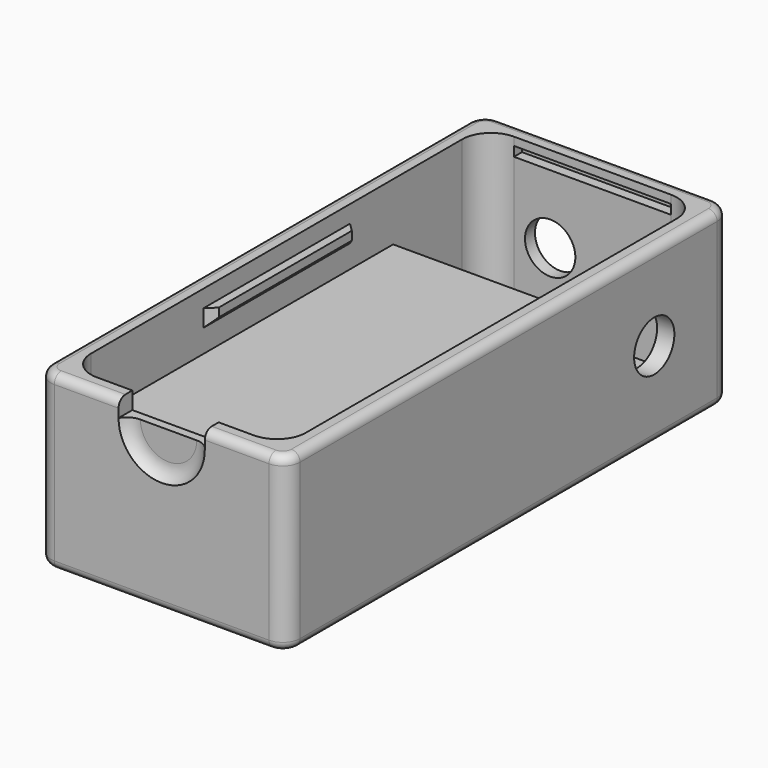
from build123d import *

# Parameters (mm, degrees)
F2_W         = 52
F2_H         = 116
F2_W_2       = 44.8
F2_H_2       = 108.8
F3_DEPTH     = 36
F4_DEPTH     = 3.6
F7_R         = 3.6
F8_R         = 5.9976
F6_R         = 5.25
F9_DEPTH     = 3.6
F5_R         = 5.25
F10_DEPTH    = 3.6
F11_W        = 18
F11_H        = 3.6
F12_DEPTH    = 3.6
F13_W        = 32.8048
F13_H        = 2
F14_DEPTH    = 2.1
F15_R        = 1.8
F6_R_2       = 12
F17_DEPTH    = 1
F18_R        = 0.5
F19_W        = 38.28
F19_H        = 3.6
F21_DEPTH    = 1.8
F20_W        = 38.28
F20_H        = 3.6
F22_DEPTH    = 1.8
F23_SIZE     = 1.79999
F25_DEPTH    = 1.8
F26_T2_ANGLE = 180
F27_W        = 41
F27_H        = 78
F28_DEPTH    = 22


# Not quite as in the source:
# - a fillet or chamfer that OpenCascade refuses, or shapes differently, is made with other operations: its cross-section is extruded or revolved along the edge and cut away or added
# - a fillet or chamfer is up to 0.001 mm smaller than in the source, because OpenCascade refuses the exact size
# - a feature of the source that left no trace in its solid (it failed there, or was rolled back) is left out


with BuildPart() as f3:
    # F2 (on Top) → F3 (new body)
    with BuildSketch(Plane.XY):
        Rectangle(F2_W, F2_H)
        Rectangle(F2_W_2, F2_H_2, mode=Mode.SUBTRACT)
    extrude(amount=F3_DEPTH)

    # F2 (on Top) → F4 (join)
    with BuildSketch(Plane.XY):
        Rectangle(F2_W_2, F2_H_2)
    extrude(amount=F4_DEPTH)

    # F7
    f7_edges = [f3.edges().sort_by_distance(p)[0] for p in [
        (26, 58, 18),
        (-26, 58, 18),
        (-26, -58, 18),
        (26, -58, 18),
    ]]
    fillet(f7_edges, radius=F7_R)

    # F8
    f8_edges = [f3.edges().sort_by_distance(p)[0] for p in [
        (-22.4, -54.4, 19.8),
        (22.4, -54.4, 19.8),
        (22.4, 54.4, 19.8),
        (-22.4, 54.4, 19.8),
    ]]
    fillet(f8_edges, radius=F8_R)

    # F6 (on face) → F9 (cut)
    with BuildSketch(Plane(origin=(0, 58, 0), x_dir=(-1, 0, 0), z_dir=(0, 1, 0))):
        with Locations((8.84, 18)):
            Circle(F6_R)
    extrude(amount=-F9_DEPTH, mode=Mode.SUBTRACT)

    # F5 (on face) → F10 (cut)
    with BuildSketch(Plane.YZ.offset(26)):
        with Locations((38, 18)):
            Circle(F5_R)
    extrude(amount=-F10_DEPTH, mode=Mode.SUBTRACT)

    # F11 (on face) → F12 (cut)
    with BuildSketch(Plane.XZ.offset(58)):
        with Locations((0, 34.2)):
            Rectangle(F11_W, F11_H)
    extrude(amount=-F12_DEPTH, mode=Mode.SUBTRACT)

    # F13 (on face) → F14 (cut)
    with BuildSketch(Plane.XZ.offset(-54.4)):
        with Locations((0, 33.3)):
            Rectangle(F13_W, F13_H)
    extrude(amount=-F14_DEPTH, mode=Mode.SUBTRACT)

    # F15
    f15_edges = [f3.edges().sort_by_distance(p)[0] for p in [
        (15.7, -58, 36),
        (24.945584, -56.945584, 36),
        (26, 0, 36),
        (-15.7, -58, 36),
        (-24.945584, -56.945584, 36),
        (-26, 0, 36),
        (-24.945584, 56.945584, 36),
        (0, 58, 36),
        (24.945584, 56.945584, 36),
        (0, -58, 0),
        (-24.945584, -56.945584, 0),
        (-26, 0, 0),
        (-24.945584, 56.945584, 0),
        (0, 58, 0),
        (24.945584, 56.945584, 0),
        (26, 0, 0),
        (24.945584, -56.945584, 0),
    ]]
    fillet(f15_edges, radius=F15_R)

    # F6 (on face) → F17 (cut)
    with BuildSketch(Plane(origin=(0, 58, 0), x_dir=(-1, 0, 0), z_dir=(0, 1, 0))):
        with Locations((8.84, 18)):
            Circle(F6_R_2)
        with Locations((8.84, 18)):
            Circle(F6_R, mode=Mode.SUBTRACT)
    extrude(amount=-F17_DEPTH, mode=Mode.SUBTRACT)

    # F18
    f18_edges = [f3.edges().sort_by_distance(p)[0] for p in [
        (0, 56.5, 34.3),
    ]]
    fillet(f18_edges, radius=F18_R)

    # F19 (on face) → F21 (join)
    with BuildSketch(Plane(origin=(22.4, 0, 0), x_dir=(0, -1, 0), z_dir=(-1, 0, 0))):
        with Locations((0, 30.6)):
            Rectangle(F19_W, F19_H)
    extrude(amount=F21_DEPTH)

    # F20 (on face) → F22 (join)
    with BuildSketch(Plane.YZ.offset(-22.4)):
        with Locations((0, 30.6)):
            Rectangle(F20_W, F20_H)
    extrude(amount=F22_DEPTH)

    # F23 (size 1.8 in the source; OpenCascade refuses exactly that, so slightly less here)
    f23_edges = [f3.edges().sort_by_distance(p)[0] for p in [
        (-20.6, -19.14, 30.6),
        (-20.6, 0, 28.8),
        (-20.6, 19.14, 30.6),
        (20.6, 19.14, 30.6),
        (20.6, 0, 28.8),
        (20.6, -19.14, 30.6),
    ]]
    chamfer(f23_edges, length=F23_SIZE)

    # F11 (on face) → F25 (cut)
    with BuildSketch(Plane.XZ.offset(58)):
        with BuildLine():
            ThreePointArc((-9, 32.4), (0, 23.4), (9, 32.4))
            Line((9, 32.4), (-9, 32.4))
        make_face()
    extrude(amount=-F25_DEPTH, mode=Mode.SUBTRACT)

    # F26: fillet of radius 3.6 on 1 edges, made by hand

    # F26_s1 → F26_t2 (revolve)
    with BuildSketch(Plane.XY.offset(32.4)):
        with BuildLine():
            ThreePointArc((-9, -58), (-7.6823085464, -56.6823085464), (-5.8823085464, -56.2))
            Line((-5.8823085464, -56.2), (-9, -56.2))
            Line((-9, -56.2), (-9, -58))
        make_face()
    revolve(axis=Axis((0, -56.2, 32.4), (0, -1, 0)), revolution_arc=F26_T2_ANGLE)


with BuildPart() as f28:
    # F27 (on face) → F28 (new body)
    with BuildSketch(Plane.XY.offset(3.6)):
        with Locations((0, -11.0006080357)):
            Rectangle(F27_W, F27_H)
    extrude(amount=F28_DEPTH)


solid = Compound([f3.part, f28.part])
